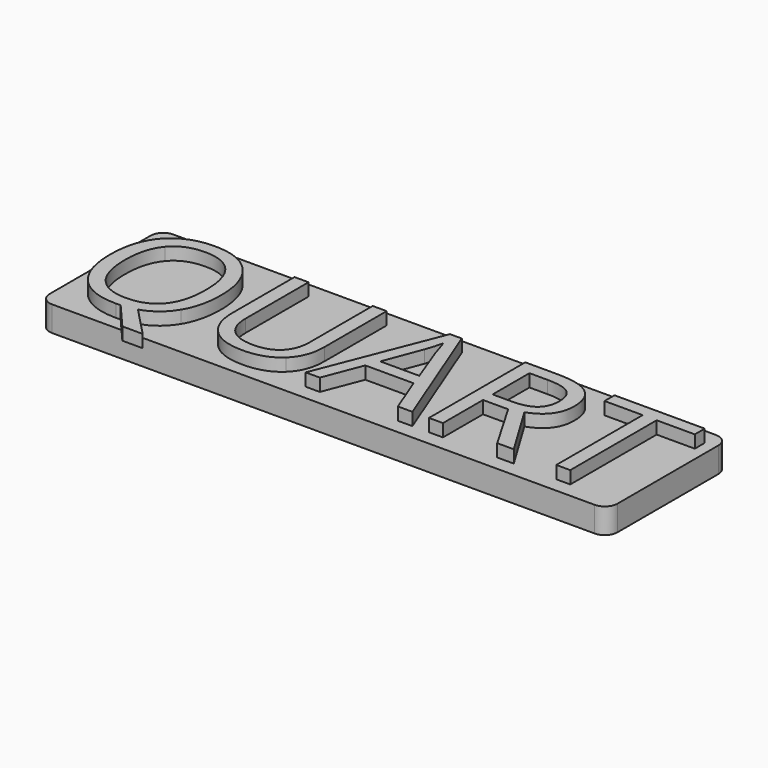
from build123d import *

# Parameters (mm, degrees)
F0_W         = 90
F0_H         = 24
F1_DEPTH     = 4
F2_R         = 2
F4_DEPTH     = 2
F5_TEXT_SIZE = 17.3611111111
F6_DEPTH     = 1.5


# Not quite as in the source:
# - a feature names something its author has since deleted; it is built from what else it names
# - Text() gives the source's letters only with a copy of the font that has no kerning and outlines rounded to 1/6400 em; it was checked with that copy


with BuildPart() as f1:
    # F0 (on Top) → F1 (new body)
    with BuildSketch(Plane.XY):
        Rectangle(F0_W, F0_H)
    extrude(amount=F1_DEPTH)

    # F2
    f2_edges = [f1.edges().sort_by_distance(p)[0] for p in [
        (-45, -12, 2),
        (45, 12, 2),
        (-45, 12, 2),
        (45, -12, 2),
    ]]
    fillet(f2_edges, radius=F2_R)

    # F3 (on face) → F4 (join)
    with BuildSketch(Plane.XY.offset(4)):
        Polygon((-26.908099327, -14.1694128568), (-28.9912722734, -12), (-32.0038858636, -12), (-30.132977489, -14.1694128568), align=None)
        with BuildLine():
            add(Edge.make_bspline(
                [(-25.8094685542, -0.0543049431), (-25.8094685542, -3.7219772569), (-27.2840566257, -6.1510791367)],
                knots=[0, 0, 0, 1, 1, 1], degree=2))
            add(Edge.make_bspline(
                [(-28.1195172894, 7.1515432815), (-25.8094685542, 4.5407287074), (-25.8094685542, -0.0543049431)],
                knots=[0, 0, 0, 1, 1, 1], degree=2))
            add(Edge.make_bspline(
                [(-34.5442097935, 9.7623578557), (-30.4295660246, 9.7623578557), (-28.1195172894, 7.1515432815)],
                knots=[0, 0, 0, 1, 1, 1], degree=2))
            add(Edge.make_bspline(
                [(-41.0691575772, 7.197493618), (-38.7716407519, 9.7623578557), (-34.5442097935, 9.7623578557)],
                knots=[0, 0, 0, 1, 1, 1], degree=2))
            add(Edge.make_bspline(
                [(-43.3666744024, -0.0292411232), (-43.3666744024, 4.6326293804), (-41.0691575772, 7.197493618)],
                knots=[0, 0, 0, 1, 1, 1], degree=2))
            add(Edge.make_bspline(
                [(-41.0754235321, -7.308192156), (-43.3666744024, -4.7287073567), (-43.3666744024, -0.0292411232)],
                knots=[0, 0, 0, 1, 1, 1], degree=2))
            add(Edge.make_bspline(
                [(-34.5692736134, -9.8876769552), (-38.7841726619, -9.8876769552), (-41.0754235321, -7.308192156)],
                knots=[0, 0, 0, 1, 1, 1], degree=2))
            Line((-34.5692736134, -9.8876769552), (-33.8507774426, -9.858435832))
            Line((-33.8507774426, -9.858435832), (-32.0038858636, -12))
            Line((-32.0038858636, -12), (-28.9912722734, -12))
            Line((-28.9912722734, -12), (-31.4488280343, -9.4407055001))
            add(Edge.make_bspline(
                [(-27.2840566257, -6.1510791367), (-28.7586446971, -8.5801810165), (-31.4488280343, -9.4407055001)],
                knots=[0, 0, 0, 1, 1, 1], degree=2))
        make_face()
        with BuildLine():
            add(Edge.make_bspline(
                [(-41.0190299373, -0.0543049431), (-41.0190299373, -3.9308424228), (-39.3669064748, -5.9359480158)],
                knots=[0, 0, 0, 1, 1, 1], degree=2))
            add(Edge.make_bspline(
                [(-39.3669064748, 5.7730331864), (-41.0190299373, 3.7679275934), (-41.0190299373, -0.0543049431)],
                knots=[0, 0, 0, 1, 1, 1], degree=2))
            add(Edge.make_bspline(
                [(-34.5442097935, 7.7781387793), (-37.7147830123, 7.7781387793), (-39.3669064748, 5.7730331864)],
                knots=[0, 0, 0, 1, 1, 1], degree=2))
            add(Edge.make_bspline(
                [(-29.7737294036, 5.787653748), (-31.3861684846, 7.7781387793), (-34.5442097935, 7.7781387793)],
                knots=[0, 0, 0, 1, 1, 1], degree=2))
            add(Edge.make_bspline(
                [(-28.1612903226, -0.0543049431), (-28.1612903226, 3.7971687166), (-29.7737294036, 5.787653748)],
                knots=[0, 0, 0, 1, 1, 1], degree=2))
            add(Edge.make_bspline(
                [(-29.7799953586, -5.9443026224), (-28.1612903226, -3.9475516361), (-28.1612903226, -0.0543049431)],
                knots=[0, 0, 0, 1, 1, 1], degree=2))
            add(Edge.make_bspline(
                [(-34.5692736134, -7.9410536087), (-31.3987003945, -7.9410536087), (-29.7799953586, -5.9443026224)],
                knots=[0, 0, 0, 1, 1, 1], degree=2))
            add(Edge.make_bspline(
                [(-39.3669064748, -5.9359480158), (-37.7147830123, -7.9410536087), (-34.5692736134, -7.9410536087)],
                knots=[0, 0, 0, 1, 1, 1], degree=2))
        make_face(mode=Mode.SUBTRACT)
        with BuildLine():
            Line((-7.1452773265, -2.8865165932), (-7.1452773265, 9.4615920167))
            Line((-7.1452773265, 9.4615920167), (-9.3634253887, 9.4615920167))
            Line((-9.3634253887, 9.4615920167), (-9.3634253887, -2.9658853562))
            add(Edge.make_bspline(
                [(-10.6688326758, -6.6544441866), (-9.3634253887, -5.3678347644), (-9.3634253887, -2.9658853562)],
                knots=[0, 0, 0, 1, 1, 1], degree=2))
            add(Edge.make_bspline(
                [(-14.388721281, -7.9410536087), (-11.9742399629, -7.9410536087), (-10.6688326758, -6.6544441866)],
                knots=[0, 0, 0, 1, 1, 1], degree=2))
            add(Edge.make_bspline(
                [(-18.2255743792, -6.6607101416), (-16.9201670921, -7.9410536087), (-14.388721281, -7.9410536087)],
                knots=[0, 0, 0, 1, 1, 1], degree=2))
            add(Edge.make_bspline(
                [(-19.5309816663, -2.9909491761), (-19.5309816663, -5.3803666744), (-18.2255743792, -6.6607101416)],
                knots=[0, 0, 0, 1, 1, 1], degree=2))
            Line((-19.5309816663, -2.9909491761), (-19.5309816663, 9.4615920167))
            Line((-19.5309816663, 9.4615920167), (-21.7533070318, 9.4615920167))
            Line((-21.7533070318, 9.4615920167), (-21.7533070318, -2.8363889534))
            add(Edge.make_bspline(
                [(-19.8672545834, -8.0058018102), (-21.7533070318, -6.1239266651), (-21.7533070318, -2.8363889534)],
                knots=[0, 0, 0, 1, 1, 1], degree=2))
            add(Edge.make_bspline(
                [(-14.5349268972, -9.8876769552), (-17.9812021351, -9.8876769552), (-19.8672545834, -8.0058018102)],
                knots=[0, 0, 0, 1, 1, 1], degree=2))
            add(Edge.make_bspline(
                [(-9.1169644929, -8.0204223718), (-11.0886516593, -9.8876769552), (-14.5349268972, -9.8876769552)],
                knots=[0, 0, 0, 1, 1, 1], degree=2))
            add(Edge.make_bspline(
                [(-7.1452773265, -2.8865165932), (-7.1452773265, -6.1531677883), (-9.1169644929, -8.0204223718)],
                knots=[0, 0, 0, 1, 1, 1], degree=2))
        make_face()
        Polygon((7.5254119285, -3.5548851242), (9.9022975168, -9.6245068461), (12.1998143421, -9.6245068461), (4.6932002785, 9.5409607798), (2.8259456951, 9.5409607798), (-4.7182640984, -9.6245068461), (-2.470874913, -9.6245068461), (-0.1232304479, -3.5548851242), align=None)
        with BuildLine():
            Line((4.6138315154, 4.3569273613), (6.8361568809, -1.5581341379))
            Line((6.8361568809, -1.5581341379), (0.662102576, -1.5581341379))
            Line((0.662102576, -1.5581341379), (2.9053144581, 4.3569273613))
            add(Edge.make_bspline(
                [(3.7282432119, 7.1097702483), (3.4400092829, 5.8565792527), (2.9053144581, 4.3569273613)],
                knots=[0, 0, 0, 1, 1, 1], degree=2))
            add(Edge.make_bspline(
                [(4.6138315154, 4.3569273613), (4.1835692736, 5.480621954), (3.7282432119, 7.1097702483)],
                knots=[0, 0, 0, 1, 1, 1], degree=2))
        make_face(mode=Mode.SUBTRACT)
        with BuildLine():
            Line((17.0413088884, -9.6245068461), (17.0413088884, -1.6876305407))
            Line((17.0413088884, -1.6876305407), (21.0264562544, -1.6876305407))
            Line((21.0264562544, -1.6876305407), (25.6465537248, -9.6245068461))
            Line((25.6465537248, -9.6245068461), (28.2699002089, -9.6245068461))
            Line((28.2699002089, -9.6245068461), (23.0858667904, -1.048503133))
            add(Edge.make_bspline(
                [(26.9248085403, 4.0686934324), (26.9248085403, 0.2840566257), (23.0858667904, -1.048503133)],
                knots=[0, 0, 0, 1, 1, 1], degree=2))
            add(Edge.make_bspline(
                [(25.2476212578, 8.1165003481), (26.9248085403, 6.7714086795), (26.9248085403, 4.0686934324)],
                knots=[0, 0, 0, 1, 1, 1], degree=2))
            add(Edge.make_bspline(
                [(20.0573218844, 9.4615920167), (23.5704339754, 9.4615920167), (25.2476212578, 8.1165003481)],
                knots=[0, 0, 0, 1, 1, 1], degree=2))
            Line((20.0573218844, 9.4615920167), (14.8231608262, 9.4615920167))
            Line((14.8231608262, 9.4615920167), (14.8231608262, -9.6245068461))
            Line((14.8231608262, -9.6245068461), (17.0413088884, -9.6245068461))
        make_face()
        with BuildLine():
            Line((20.0865630077, 0.2172197726), (17.0413088884, 0.2172197726))
            Line((17.0413088884, 0.2172197726), (17.0413088884, 7.5149686702))
            Line((17.0413088884, 7.5149686702), (19.9278254816, 7.5149686702))
            add(Edge.make_bspline(
                [(23.5119517289, 6.6795080065), (22.3966117429, 7.5149686702), (19.9278254816, 7.5149686702)],
                knots=[0, 0, 0, 1, 1, 1], degree=2))
            add(Edge.make_bspline(
                [(24.627291715, 3.9517289394), (24.627291715, 5.8440473428), (23.5119517289, 6.6795080065)],
                knots=[0, 0, 0, 1, 1, 1], degree=2))
            add(Edge.make_bspline(
                [(23.5307495939, 1.1508470643), (24.627291715, 2.084474356), (24.627291715, 3.9517289394)],
                knots=[0, 0, 0, 1, 1, 1], degree=2))
            add(Edge.make_bspline(
                [(20.0865630077, 0.2172197726), (22.4342074727, 0.2172197726), (23.5307495939, 1.1508470643)],
                knots=[0, 0, 0, 1, 1, 1], degree=2))
        make_face(mode=Mode.SUBTRACT)
        Polygon((35.0037131585, -9.6245068461), (37.2218612207, -9.6245068461), (37.2218612207, 7.4899048503), (43.2664191228, 7.4899048503), (43.2664191228, 9.4615920167), (28.9591552564, 9.4615920167), (28.9591552564, 7.4899048503), (35.0037131585, 7.4899048503), align=None)
    extrude(amount=F4_DEPTH)

    # F5 (on face) → F6 (cut)
    with BuildSketch(Plane(origin=(0, 0, 0), x_dir=(1, 0, 0), z_dir=(0, 0, -1))):
        with Locations((-27.4305555556, -6.25)):
            Text('2 pints', F5_TEXT_SIZE, font='Open Sans', text_align=(TextAlign.LEFT, TextAlign.BOTTOM))
    extrude(amount=-F6_DEPTH, mode=Mode.SUBTRACT)


solid = f1.part
